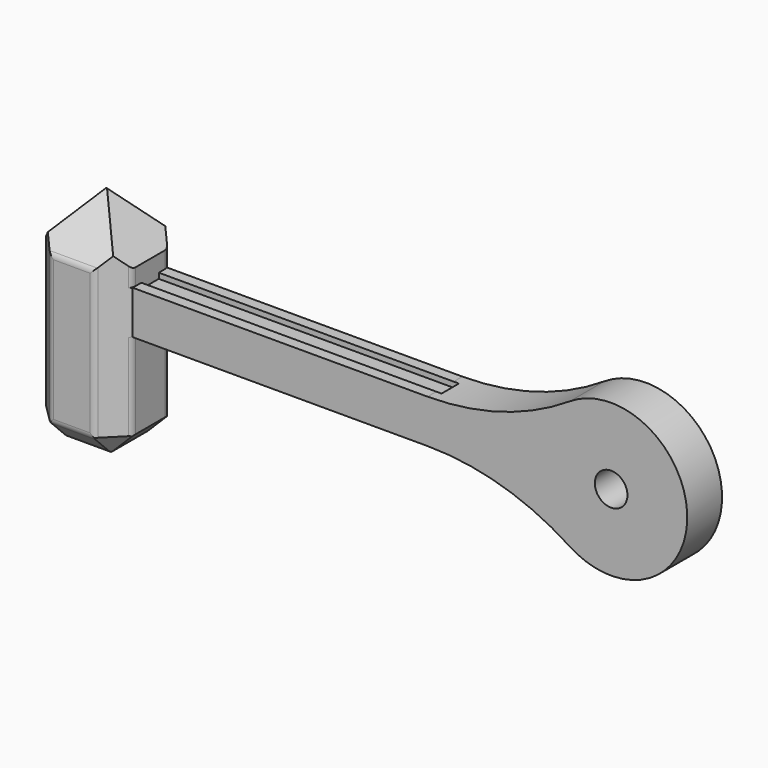
from build123d import *

# Parameters (mm, degrees)
F0_R          = 19.05
F1_DEPTH      = 50.8
F2_W          = 101.6
F2_H          = 254
F3_DEPTH      = 101.6
F5_DEPTH      = 150.00483
F7_DEPTH      = 133.96625
F8_SIZE       = 25.39999
F9_T1_DEPTH   = 70.526940908
F9_T3_DEPTH   = 70.526940908
F10_T1_DEPTH  = 69.1227672529
F10_T3_DEPTH  = 191.4591513789
F10_T5_DEPTH  = 70.526940908
F10_T7_DEPTH  = 68.974059705
F10_T9_DEPTH  = 70.526940908
F11_T4_DEPTH  = 191.4591513789
F11_T9_DEPTH  = 191.4591513789
F11_T14_DEPTH = 191.4591513789
F11_T19_DEPTH = 191.4591513789
F13_R         = 12.7
F14_DEPTH     = 159.81291
F15_W         = 344.3993236951
F15_H         = 25.4
F16_DEPTH     = 6.35
F17_W         = 344.3993236951
F17_H         = 25.4
F18_DEPTH     = 6.35
F19_T1_DEPTH  = 25.4
F21_DEPTH     = 157.5482


# Not quite as in the source:
# - a fillet or chamfer that OpenCascade refuses, or shapes differently, is made with other operations: its cross-section is extruded or revolved along the edge and cut away or added
# - a fillet or chamfer is up to 0.001 mm smaller than in the source, because OpenCascade refuses the exact size
# - a feature of the source that left no trace in its solid (it failed there, or was rolled back) is left out


with BuildPart() as f1:
    # F0 (on Front) → F1 (new body)
    with BuildSketch(Plane.XZ):
        with BuildLine():
            ThreePointArc((-214.4006763049, -25.4), (-127.8432927657, -37.9486366929), (-48.4130559398, -74.5612903226))
            ThreePointArc((-48.4130559398, -74.5612903226), (88.9, 0), (-48.4130559398, 74.5612903226))
            ThreePointArc((-48.4130559398, 74.5612903226), (-127.8432927657, 37.9486366929), (-214.4006763049, 25.4))
            Line((-214.4006763049, 25.4), (-558.8, 25.4))
            Line((-558.8, 25.4), (-558.8, -25.4))
            Line((-558.8, -25.4), (-214.4006763049, -25.4))
        make_face()
        Circle(F0_R, mode=Mode.SUBTRACT)
    extrude(amount=F1_DEPTH)

    # F2 (on face) → F3 (join)
    with BuildSketch(Plane(origin=(-558.8, 0, 0), x_dir=(0, -1, 0), z_dir=(-1, 0, 0))):
        with Locations((25.4, -25.4)):
            Rectangle(F2_W, F2_H)
    extrude(amount=F3_DEPTH)

    # F4 (on face) → F5 (cut)
    with BuildSketch(Plane(origin=(0, 25.4, 0), x_dir=(-1, 0, 0), z_dir=(0, 1, 0))):
        Polygon((534.5858503342, 124.7548833489), (558.8, 44.7322204709), (609.6, 101.6), (660.4, 44.7322204709), (660.4, 124.7548833489), align=None)
    extrude(amount=-F5_DEPTH, mode=Mode.SUBTRACT)

    # F6 (on face) → F7 (cut)
    with BuildSketch(Plane(origin=(-660.4, 0, 0), x_dir=(0, -1, 0), z_dir=(-1, 0, 0))):
        Polygon((-36.009144038, 107.4853688478), (-25.4, 44.7322204709), (25.4, 100.9804829955), (76.2, 44.7322204709), (85.7249945402, 107.4853688478), align=None)
    extrude(amount=-F7_DEPTH, mode=Mode.SUBTRACT)

    # F8 (size 25.4 in the source; OpenCascade refuses exactly that, so slightly less here)
    f8_edges = [f1.edges().sort_by_distance(p)[0] for p in [
        (-660.4, -76.2, -53.83389),
        (-558.8, -76.2, -53.83389),
        (-558.8, 25.4, -53.83389),
        (-660.4, 25.4, -53.83389),
        (-609.6, 25.4, -152.4),
        (-609.6, -76.2, -152.4),
        (-558.8, -25.4, -152.4),
        (-660.4, -25.4, -152.4),
    ]]
    chamfer(f8_edges, length=F8_SIZE)

    # F9: fillet of radius 9.525 on 4 edges, made by hand

    # F9_s2 → F9_t1 (cut)
    with BuildSketch(Plane.YZ.offset(-644.863470454)):
        with BuildLine():
            ThreePointArc((2.7898179092, -149.6101920908), (-0.3003144883, -151.6749525472), (-3.9453741816, -152.4))
            Line((-3.9453741816, -152.4), (1e-05, -152.4))
            Line((1e-05, -152.4), (2.7898179092, -149.6101920908))
        make_face()
        with BuildLine():
            ThreePointArc((-53.5898179092, -149.6101920908), (-50.4996855117, -151.6749525472), (-46.8546258184, -152.4))
            Line((-46.8546258184, -152.4), (-50.80001, -152.4))
            Line((-50.80001, -152.4), (-53.5898179092, -149.6101920908))
        make_face()
    extrude(amount=F9_T1_DEPTH, mode=Mode.SUBTRACT)

    # F9_s4 → F9_t3 (cut)
    with BuildSketch(Plane.XZ.offset(-9.863470454)):
        with BuildLine():
            ThreePointArc((-581.4101820908, -149.6101920908), (-584.5003144883, -151.6749525472), (-588.1453741816, -152.4))
            Line((-588.1453741816, -152.4), (-584.19999, -152.4))
            Line((-584.19999, -152.4), (-581.4101820908, -149.6101920908))
        make_face()
        with BuildLine():
            ThreePointArc((-631.0546258184, -152.4), (-634.6996855117, -151.6749525472), (-637.7898179092, -149.6101920908))
            Line((-637.7898179092, -149.6101920908), (-635.00001, -152.4))
            Line((-635.00001, -152.4), (-631.0546258184, -152.4))
        make_face()
    extrude(amount=F9_T3_DEPTH, mode=Mode.SUBTRACT)

    # F10: fillet of radius 9.525 on 12 edges, made by hand

    # F10_s2 → F10_t1 (cut)
    with BuildSketch(Plane.YZ.offset(-644.1613836265)):
        with BuildLine():
            ThreePointArc((-73.7438328649, 47.4518097193), (-75.5647766574, 44.4878312477), (-76.2, 41.0676710203))
            Line((-76.2, 41.0676710203), (-76.2, 44.7322204709))
            Line((-76.2, 44.7322204709), (-73.7438328649, 47.4518097193))
        make_face()
        with BuildLine():
            ThreePointArc((22.9438328649, 47.4518097193), (24.7647766574, 44.4878312477), (25.4, 41.0676710203))
            Line((25.4, 41.0676710203), (25.4, 44.7322204709))
            Line((25.4, 44.7322204709), (22.9438328649, 47.4518097193))
        make_face()
    extrude(amount=F10_T1_DEPTH, mode=Mode.SUBTRACT)

    # F10_s4 → F10_t3 (cut)
    with BuildSketch(Plane.XY.offset(-136.863470454)):
        with BuildLine():
            ThreePointArc((-637.7898179092, -73.4101920908), (-634.6996855117, -75.4749525472), (-631.0546258184, -76.2))
            Line((-631.0546258184, -76.2), (-635.00001, -76.2))
            Line((-635.00001, -76.2), (-637.7898179092, -73.4101920908))
        make_face()
        with BuildLine():
            ThreePointArc((-581.4101820908, -73.4101920908), (-584.5003144883, -75.4749525472), (-588.1453741816, -76.2))
            Line((-588.1453741816, -76.2), (-584.19999, -76.2))
            Line((-584.19999, -76.2), (-581.4101820908, -73.4101920908))
        make_face()
        with BuildLine():
            ThreePointArc((-637.7898179092, 22.6101920908), (-634.6996855117, 24.6749525472), (-631.0546258184, 25.4))
            Line((-631.0546258184, 25.4), (-635.00001, 25.4))
            Line((-635.00001, 25.4), (-637.7898179092, 22.6101920908))
        make_face()
        with BuildLine():
            ThreePointArc((-581.4101820908, 22.6101920908), (-584.5003144883, 24.6749525472), (-588.1453741816, 25.4))
            Line((-588.1453741816, 25.4), (-584.19999, 25.4))
            Line((-584.19999, 25.4), (-581.4101820908, 22.6101920908))
        make_face()
        with BuildLine():
            ThreePointArc((-657.6101920908, 2.7898179092), (-659.6749525472, -0.3003144883), (-660.4, -3.9453741816))
            Line((-660.4, -3.9453741816), (-660.4, 1e-05))
            Line((-660.4, 1e-05), (-657.6101920908, 2.7898179092))
        make_face()
        with BuildLine():
            ThreePointArc((-657.6101920908, -53.5898179092), (-659.6749525472, -50.4996855117), (-660.4, -46.8546258184))
            Line((-660.4, -46.8546258184), (-660.4, -50.80001))
            Line((-660.4, -50.80001), (-657.6101920908, -53.5898179092))
        make_face()
    extrude(amount=F10_T3_DEPTH, mode=Mode.SUBTRACT)

    # F10_s6 → F10_t5 (cut)
    with BuildSketch(Plane.YZ.offset(-644.863470454)):
        with BuildLine():
            ThreePointArc((-76.2, -123.0546258184), (-75.4749525472, -126.6996855117), (-73.4101920908, -129.7898179092))
            Line((-73.4101920908, -129.7898179092), (-76.2, -127.00001))
            Line((-76.2, -127.00001), (-76.2, -123.0546258184))
        make_face()
        with BuildLine():
            ThreePointArc((25.4, -123.0546258184), (24.6749525472, -126.6996855117), (22.6101920908, -129.7898179092))
            Line((22.6101920908, -129.7898179092), (25.4, -127.00001))
            Line((25.4, -127.00001), (25.4, -123.0546258184))
        make_face()
    extrude(amount=F10_T5_DEPTH, mode=Mode.SUBTRACT)

    # F10_s8 → F10_t7 (cut)
    with BuildSketch(Plane.XZ.offset(-9.0870298525)):
        with BuildLine():
            ThreePointArc((-657.9784923634, 47.4429638254), (-659.7740558421, 44.4933557154), (-660.4, 41.0974125299))
            Line((-660.4, 41.0974125299), (-660.4, 44.7322204709))
            Line((-660.4, 44.7322204709), (-657.9784923634, 47.4429638254))
        make_face()
    extrude(amount=F10_T7_DEPTH, mode=Mode.SUBTRACT)

    # F10_s10 → F10_t9 (cut)
    with BuildSketch(Plane.XZ.offset(-9.863470454)):
        with BuildLine():
            ThreePointArc((-660.4, -123.0546258184), (-659.6749525472, -126.6996855117), (-657.6101920908, -129.7898179092))
            Line((-657.6101920908, -129.7898179092), (-660.4, -127.00001))
            Line((-660.4, -127.00001), (-660.4, -123.0546258184))
        make_face()
    extrude(amount=F10_T9_DEPTH, mode=Mode.SUBTRACT)

    # F11: fillet of radius 9.525 on 2 edges, made by hand


with BuildPart() as f11_tool2:
    # F11_s3 → F11_t4 (new body)
    with BuildSketch(Plane.XY.offset(-136.863470454)):
        with BuildLine():
            ThreePointArc((-558.8, -46.8546258184), (-559.5250474528, -50.4996855117), (-561.5898079092, -53.5898179092))
            Line((-561.5898079092, -53.5898179092), (-558.8, -50.80001))
            Line((-558.8, -50.80001), (-558.8, -46.8546258184))
        make_face()
    extrude(amount=F11_T4_DEPTH)

    split(bisect_by=Plane.XY.offset(-25.4), keep=Keep.BOTTOM)


with BuildPart() as f1_1:
    add(f1.part)

    # F11_t1: cut F11_tool2
    add(f11_tool2.part, mode=Mode.SUBTRACT)


with BuildPart() as f11_tool7:
    # F11_s8 → F11_t9 (new body)
    with BuildSketch(Plane.XY.offset(-136.863470454)):
        with BuildLine():
            ThreePointArc((-558.8, -46.8546258184), (-559.5250474528, -50.4996855117), (-561.5898079092, -53.5898179092))
            Line((-561.5898079092, -53.5898179092), (-558.8, -50.80001))
            Line((-558.8, -50.80001), (-558.8, -46.8546258184))
        make_face()
    extrude(amount=F11_T9_DEPTH)

    split(bisect_by=Plane.XY.offset(25.4), keep=Keep.TOP)


with BuildPart() as f1_2:
    add(f1_1.part)

    # F11_t6: cut F11_tool7
    add(f11_tool7.part, mode=Mode.SUBTRACT)


with BuildPart() as f11_tool12:
    # F11_s13 → F11_t14 (new body)
    with BuildSketch(Plane.XY.offset(54.5956809249)):
        with BuildLine():
            ThreePointArc((-561.5898079092, 2.7898179092), (-559.5250474528, -0.3003144883), (-558.8, -3.9453741816))
            Line((-558.8, -3.9453741816), (-558.8, 1e-05))
            Line((-558.8, 1e-05), (-561.5898079092, 2.7898179092))
        make_face()
    extrude(amount=-F11_T14_DEPTH)

    split(bisect_by=Plane.XY.offset(25.4), keep=Keep.TOP)


with BuildPart() as f1_3:
    add(f1_2.part)

    # F11_t11: cut F11_tool12
    add(f11_tool12.part, mode=Mode.SUBTRACT)


with BuildPart() as f11_tool17:
    # F11_s18 → F11_t19 (new body)
    with BuildSketch(Plane.XY.offset(54.5956809249)):
        with BuildLine():
            ThreePointArc((-561.5898079092, 2.7898179092), (-559.5250474528, -0.3003144883), (-558.8, -3.9453741816))
            Line((-558.8, -3.9453741816), (-558.8, 1e-05))
            Line((-558.8, 1e-05), (-561.5898079092, 2.7898179092))
        make_face()
    extrude(amount=-F11_T19_DEPTH)

    split(bisect_by=Plane.XY.offset(-25.4), keep=Keep.BOTTOM)


with BuildPart() as f1_4:
    add(f1_3.part)

    # F11_t16: cut F11_tool17
    add(f11_tool17.part, mode=Mode.SUBTRACT)

    # F13 (on face) → F14 (cut)
    with BuildSketch(Plane(origin=(0, 0, -152.4), x_dir=(1, 0, 0), z_dir=(0, 0, -1))):
        with Locations((-609.6, 25.4)):
            Circle(F13_R)
    extrude(amount=-F14_DEPTH, mode=Mode.SUBTRACT)

    # F15 (on face) → F16 (cut)
    with BuildSketch(Plane.XY.offset(25.4)):
        with Locations((-386.6003381525, -25.4)):
            Rectangle(F15_W, F15_H)
    extrude(amount=-F16_DEPTH, mode=Mode.SUBTRACT)

    # F17 (on face) → F18 (cut)
    with BuildSketch(Plane(origin=(0, 0, -25.4), x_dir=(1, 0, 0), z_dir=(0, 0, -1))):
        with Locations((-386.6003381525, 25.4)):
            Rectangle(F17_W, F17_H)
    extrude(amount=-F18_DEPTH, mode=Mode.SUBTRACT)

    # F19: chamfer of 6.35 on 6 edges, made by hand

    # F19_s2 → F19_t1 (cut)
    with BuildSketch(Plane.XZ.offset(12.7)):
        with BuildLine():
            Line((-208.1802681416, -25.4634801631), (-214.4006763049, -19.1148026665))
            Line((-214.4006763049, -19.1148026665), (-214.4006763049, -25.4))
            ThreePointArc((-214.4006763049, -25.4), (-211.2004813817, -25.4168004098), (-208.1802681416, -25.4634801631))
        make_face()
        with BuildLine():
            Line((-208.1802681416, 25.4634801631), (-214.4006763049, 19.1148026665))
            Line((-214.4006763049, 19.1148026665), (-214.4006763049, 25.4))
            ThreePointArc((-214.4006763049, 25.4), (-211.2004813817, 25.4168004098), (-208.1802681416, 25.4634801631))
        make_face()
    extrude(amount=F19_T1_DEPTH, mode=Mode.SUBTRACT)

    # F20 (on face) → F21 (join)
    with BuildSketch(Plane(origin=(0, 0, 7.41291), x_dir=(1, 0, 0), z_dir=(0, 0, -1))):
        Polygon((-613.0348443985, 25.984024629), (-626.3800263405, 31.7753516138), (-628.3944249153, 25.984024629), align=None)
        Polygon((-591.8838977814, 23.9696521312), (-606.2363386154, 24.2214500904), (-591.8838977814, 17.4229387194), align=None)
    extrude(amount=F21_DEPTH)


solid = f1_4.part
